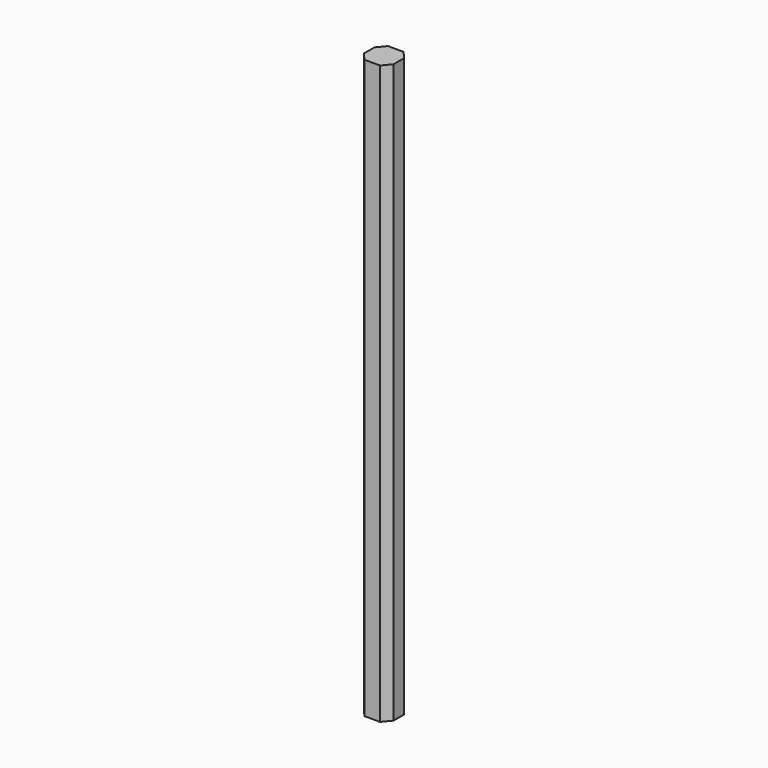
from build123d import *

# Parameters (mm, degrees)
F1_DEPTH = 762


# Not quite as in the source:
# - a feature of the source that left no trace in its solid (it failed there, or was rolled back) is left out
# - a pattern or mirror of a feature is missing from the dataset's text; its kind, count and spacing are read off the source's solid


with BuildPart() as f1:
    # F0 (on Top) → F1 (new body)
    with BuildSketch(Plane.XY):
        Polygon((-29.8925630746, 10.9454181869), (-39, 0), (-39, -17.1091636262), (-29.8925630746, -28.0545818131), (-9.1074369254, -28.0545818131), (0, -17.1091636262), (0, 0), (-9.1074369254, 10.9454181869), align=None)
    extrude(amount=F1_DEPTH)

    # F1_copies: F1 across plane


with BuildPart() as f1_1:
    add(f1.part)
    add(f1.part.mirror(Plane.XY.offset(382.001728)))


solid = f1_1.part
